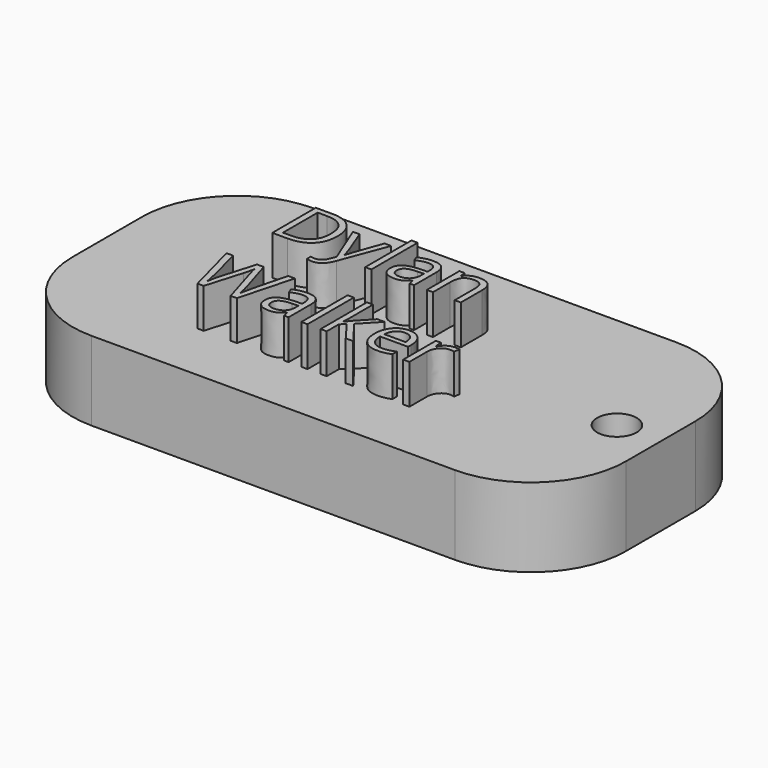
from build123d import *

# Parameters (mm, degrees)
F0_W         = 70
F0_H         = 35
F1_DEPTH     = 10
F2_R         = 12
F5_D         = 5
F3_TEXT_SIZE = 9.6286106984
F6_DEPTH     = 5


# Not quite as in the source:
# - Text() gives the source's letters only with a copy of the font that has no kerning and outlines rounded to 1/6400 em; it was checked with that copy


with BuildPart() as f1:
    # F0 (on Top) → F1 (new body)
    with BuildSketch(Plane.XY):
        with Locations((2.5997259654, 0)):
            Rectangle(F0_W, F0_H)
    extrude(amount=F1_DEPTH)

    # F2
    f2_edges = [f1.edges().sort_by_distance(p)[0] for p in [
        (37.599726, -17.5, 5),
        (37.599726, 17.5, 5),
        (-32.400274, -17.5, 5),
        (-32.400274, 17.5, 5),
    ]]
    fillet(f2_edges, radius=F2_R)

    # F5 (through all)
    with Locations(Plane(origin=(0, 0, 0), x_dir=(1, 0, 0), z_dir=(0, 0, -1))):
        with Locations((32.0632755756, 0)):
            Hole(F5_D / 2)

    # F3 (on face) → F6 (join)
    with BuildSketch(Plane.XY.offset(10)):
        with Locations((-15.1650621556, 3.3579801675)):
            Text('Dylan', F3_TEXT_SIZE, font='Open Sans', text_align=(TextAlign.LEFT, TextAlign.BOTTOM))
        with Locations((-15.1650621556, -9.7369303823)):
            Text('Walker', F3_TEXT_SIZE, font='Open Sans', text_align=(TextAlign.LEFT, TextAlign.BOTTOM))
    extrude(amount=F6_DEPTH)


solid = f1.part
